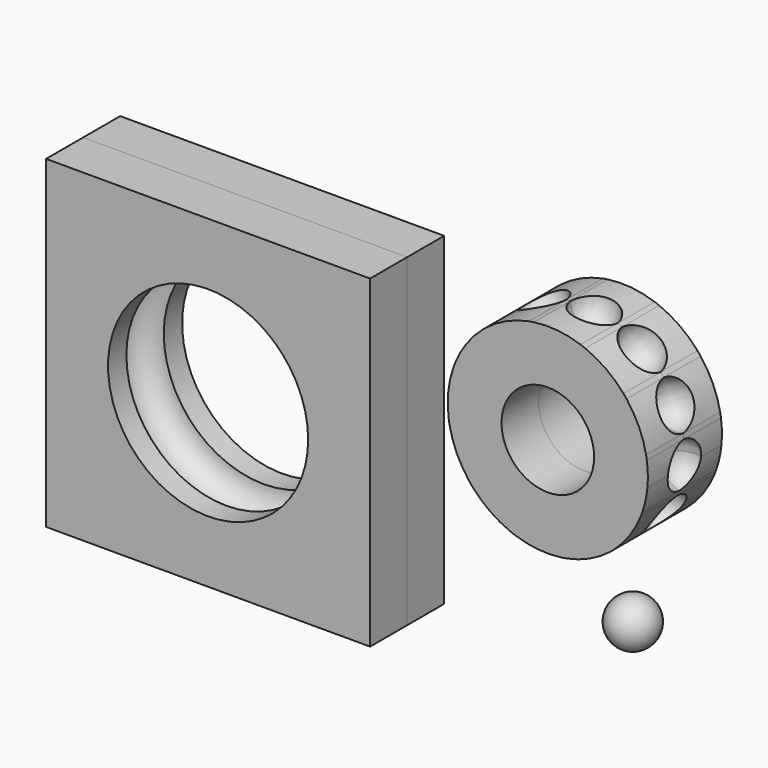
from build123d import *
from build123d import SkipClean  # not in build123d's __all__

# Parameters (mm, degrees)
F2_W      = 88.9
F2_H      = 88.9
F2_R      = 27.45
F5_DEPTH  = 12.7
F4_R      = 6.41
F7_R      = 12.7
F8_DEPTH  = 12.7
F22_W     = 3.2742018811
F22_H     = 5.4303631186
F23_DEPTH = 0.1
F22_R     = 2.7331759806
F24_DEPTH = 0.1


with BuildPart() as f1:
    # F0 (on Front) → F1 (revolve)
    with BuildSketch(Plane.XZ):
        with BuildLine():
            Line((0, 6.5), (0, -6.5))
            ThreePointArc((0, -6.5), (6.5, 0), (0, 6.5))
        make_face()
    revolve(axis=Axis((0, 0, 0), (0, 0, -1)))


with BuildPart() as f5:
    # F2 (on Front) → F5 (new body)
    with BuildSketch(Plane.XZ):
        with Locations((-106.35, 23.4373745618)):
            Rectangle(F2_W, F2_H)
        with Locations((-106.35, 23.4373745618)):
            Circle(F2_R, mode=Mode.SUBTRACT)
    extrude(amount=F5_DEPTH)

    # F4 (on face) → F6 (revolve, cut)
    with BuildSketch(Plane(origin=(0, 0, 23.4373745618), x_dir=(1, 0, 0), z_dir=(0, 0, -1))):
        with Locations((-133.8, 0)):
            Circle(F4_R)
    revolve(axis=Axis((-106.35, 0, 23.4373745618), (0, -1, 0)), mode=Mode.SUBTRACT)

    # F25: F5 across face


with BuildPart() as f8:
    # F7 (on Front) → F8 (new body)
    with BuildSketch(Plane.XZ):
        with BuildLine():
            Line((13.4063024508, 42.210689718), (14.0268309363, 48.6350721316))
            ThreePointArc((14.0268309363, 48.6350721316), (9.7490674331, 46.8995620632), (7.7024290215, 42.7616245336))
            Line((7.7024290215, 42.7616245336), (13.4063024508, 42.210689718))
        make_face()
        with BuildLine():
            Line((13.4063024508, 42.210689718), (7.7024290215, 42.7616245336))
            ThreePointArc((7.7024290215, 42.7616245336), (8.9192573509, 38.3084700783), (12.7857739652, 35.7863073044))
            Line((12.7857739652, 35.7863073044), (13.4063024508, 42.210689718))
        make_face()
        with BuildLine():
            ThreePointArc((14.1723185105, 42.1367005382), (14.2676693344, 43.4547207628), (14.2994775146, 44.7758026421))
            ThreePointArc((14.2994775146, 44.7758026421), (14.2312310325, 46.7102468225), (14.0268309363, 48.6350721316))
            Line((14.0268309363, 48.6350721316), (13.4063024508, 42.210689718))
            Line((13.4063024508, 42.210689718), (14.1723185105, 42.1367005382))
        make_face()
        with BuildLine():
            ThreePointArc((12.7857739652, 35.7863073044), (13.6676766328, 38.9203183702), (14.1723185105, 42.1367005382))
            Line((14.1723185105, 42.1367005382), (13.4063024508, 42.210689718))
            Line((13.4063024508, 42.210689718), (12.7857739652, 35.7863073044))
        make_face()
        with BuildLine():
            Line((8.4561212407, 61.7067047709), (13.8057167898, 49.9588195377))
            ThreePointArc((13.8057167898, 49.9588195377), (11.8313029726, 56.1516936749), (8.4561212407, 61.7067047709))
        make_face()
        with BuildLine():
            Line((-2.9040711925, 70.2417158577), (7.6027570696, 62.7425465795))
            ThreePointArc((7.6027570696, 62.7425465795), (2.7964274777, 67.1185259961), (-2.9040711925, 70.2417158577))
        make_face()
        with BuildLine():
            ThreePointArc((8.4561212407, 61.7067047709), (5.9157523177, 53.4579489859), (13.8057167898, 49.9588195377))
            Line((13.8057167898, 49.9588195377), (8.4561212407, 61.7067047709))
        make_face()
        with BuildLine():
            ThreePointArc((-2.9040711925, 70.2417158577), (-0.9797173223, 61.8278993367), (7.6027570696, 62.7425465795))
            Line((7.6027570696, 62.7425465795), (-2.9040711925, 70.2417158577))
        make_face()
        with BuildLine():
            ThreePointArc((-17.0097919748, 71.9531560638), (-11.1363443769, 65.628754149), (-4.1610271476, 70.7120990927))
            Line((-4.1610271476, 70.7120990927), (-17.0097919748, 71.9531560638))
        make_face()
        with BuildLine():
            ThreePointArc((-30.0814246141, 66.3824463682), (-21.8326688291, 63.8420774452), (-18.333539381, 71.7320419173))
            Line((-18.333539381, 71.7320419173), (-30.0814246141, 66.3824463682))
        make_face()
        with BuildLine():
            ThreePointArc((-38.6164357009, 55.022253935), (-30.20261918, 56.9466078052), (-31.1172664228, 65.5290821971))
            Line((-31.1172664228, 65.5290821971), (-38.6164357009, 55.022253935))
        make_face()
        with BuildLine():
            ThreePointArc((7.7024290215, 42.7616245336), (9.7490674331, 46.8995620632), (14.0268309363, 48.6350721316))
            ThreePointArc((14.0268309363, 48.6350721316), (13.9243651666, 49.2982973777), (13.8057167898, 49.9588195377))
            ThreePointArc((13.8057167898, 49.9588195377), (5.9157523177, 53.4579489859), (8.4561212407, 61.7067047709))
            ThreePointArc((8.4561212407, 61.7067047709), (8.035770658, 62.2298417976), (7.6027570696, 62.7425465795))
            ThreePointArc((7.6027570696, 62.7425465795), (-0.9797173223, 61.8278993367), (-2.9040711925, 70.2417158577))
            ThreePointArc((-2.9040711925, 70.2417158577), (-3.5296739889, 70.4845905211), (-4.1610271476, 70.7120990927))
            ThreePointArc((-4.1610271476, 70.7120990927), (-11.1363443769, 65.628754149), (-17.0097919748, 71.9531560638))
            ThreePointArc((-17.0097919748, 71.9531560638), (-17.673017221, 71.8506902941), (-18.333539381, 71.7320419173))
            ThreePointArc((-18.333539381, 71.7320419173), (-21.8326688291, 63.8420774452), (-30.0814246141, 66.3824463682))
            ThreePointArc((-30.0814246141, 66.3824463682), (-30.6045616409, 65.9620957855), (-31.1172664228, 65.5290821971))
            ThreePointArc((-31.1172664228, 65.5290821971), (-30.20261918, 56.9466078052), (-38.6164357009, 55.022253935))
            ThreePointArc((-38.6164357009, 55.022253935), (-38.8593103644, 54.3966511385), (-39.086818936, 53.7652979798))
            ThreePointArc((-39.086818936, 53.7652979798), (-34.0034739922, 46.7899807506), (-40.3278759071, 40.9165331526))
            ThreePointArc((-40.3278759071, 40.9165331526), (-40.2254101373, 40.2533079065), (-40.1067617605, 39.5927857465))
            ThreePointArc((-40.1067617605, 39.5927857465), (-32.2167972884, 36.0936562984), (-34.7571662115, 27.8449005133))
            ThreePointArc((-34.7571662115, 27.8449005133), (-34.3368156288, 27.3217634866), (-33.9038020403, 26.8090587047))
            ThreePointArc((-33.9038020403, 26.8090587047), (-25.3213276485, 27.7237059475), (-23.3969737783, 19.3098894266))
            ThreePointArc((-23.3969737783, 19.3098894266), (-22.7713709818, 19.0670147631), (-22.1400178231, 18.8395061915))
            ThreePointArc((-22.1400178231, 18.8395061915), (-15.1647005938, 23.9228511352), (-9.2912529959, 17.5984492204))
            ThreePointArc((-9.2912529959, 17.5984492204), (-8.6280277497, 17.7009149901), (-7.9675055898, 17.8195633669))
            ThreePointArc((-7.9675055898, 17.8195633669), (-4.4683761416, 25.7095278391), (3.7803796434, 23.169158916))
            ThreePointArc((3.7803796434, 23.169158916), (4.3035166702, 23.5895094987), (4.8162214521, 24.0225230871))
            ThreePointArc((4.8162214521, 24.0225230871), (3.9015742092, 32.604997479), (12.3153907302, 34.5293513492))
            ThreePointArc((12.3153907302, 34.5293513492), (12.5582653936, 35.1549541457), (12.7857739652, 35.7863073044))
            ThreePointArc((12.7857739652, 35.7863073044), (8.9192573509, 38.3084700783), (7.7024290215, 42.7616245336))
        make_face()
        with Locations((-13.1505224854, 44.7758026421)):
            Circle(F7_R, mode=Mode.SUBTRACT)
        with BuildLine():
            Line((4.8162214521, 24.0225230871), (12.3153907302, 34.5293513492))
            ThreePointArc((12.3153907302, 34.5293513492), (3.9015742092, 32.604997479), (4.8162214521, 24.0225230871))
        make_face()
        with BuildLine():
            Line((-7.9675055898, 17.8195633669), (3.7803796434, 23.169158916))
            ThreePointArc((3.7803796434, 23.169158916), (-4.4683761416, 25.7095278391), (-7.9675055898, 17.8195633669))
        make_face()
        with BuildLine():
            Line((-22.1400178231, 18.8395061915), (-9.2912529959, 17.5984492204))
            ThreePointArc((-9.2912529959, 17.5984492204), (-15.1647005938, 23.9228511352), (-22.1400178231, 18.8395061915))
        make_face()
        with BuildLine():
            Line((-33.9038020403, 26.8090587047), (-23.3969737783, 19.3098894266))
            ThreePointArc((-23.3969737783, 19.3098894266), (-25.3213276485, 27.7237059475), (-33.9038020403, 26.8090587047))
        make_face()
        with BuildLine():
            Line((-40.1067617605, 39.5927857465), (-34.7571662115, 27.8449005133))
            ThreePointArc((-34.7571662115, 27.8449005133), (-32.2167972884, 36.0936562984), (-40.1067617605, 39.5927857465))
        make_face()
        with BuildLine():
            ThreePointArc((-40.3278759071, 40.9165331526), (-34.0034739922, 46.7899807506), (-39.086818936, 53.7652979798))
            Line((-39.086818936, 53.7652979798), (-40.3278759071, 40.9165331526))
        make_face()
        with BuildLine():
            Line((-30.0814246141, 66.3824463682), (-18.333539381, 71.7320419173))
            ThreePointArc((-18.333539381, 71.7320419173), (-24.5264135181, 69.7576281), (-30.0814246141, 66.3824463682))
        make_face()
        with BuildLine():
            Line((-38.6164357009, 55.022253935), (-31.1172664228, 65.5290821971))
            ThreePointArc((-31.1172664228, 65.5290821971), (-35.4932458394, 60.7227526052), (-38.6164357009, 55.022253935))
        make_face()
        with BuildLine():
            Line((-17.0097919748, 71.9531560638), (-4.1610271476, 70.7120990927))
            ThreePointArc((-4.1610271476, 70.7120990927), (-10.5114203815, 72.098643638), (-17.0097919748, 71.9531560638))
        make_face()
        with BuildLine():
            Line((-40.3278759071, 40.9165331526), (-39.086818936, 53.7652979798))
            ThreePointArc((-39.086818936, 53.7652979798), (-40.4733634812, 47.414904746), (-40.3278759071, 40.9165331526))
        make_face()
        with BuildLine():
            ThreePointArc((-40.1067617605, 39.5927857465), (-38.1323479433, 33.3999116094), (-34.7571662115, 27.8449005133))
            Line((-34.7571662115, 27.8449005133), (-40.1067617605, 39.5927857465))
        make_face()
        with BuildLine():
            ThreePointArc((-33.9038020403, 26.8090587047), (-29.0974724485, 22.4330792881), (-23.3969737783, 19.3098894266))
            Line((-23.3969737783, 19.3098894266), (-33.9038020403, 26.8090587047))
        make_face()
        with BuildLine():
            ThreePointArc((-22.1400178231, 18.8395061915), (-15.7896245893, 17.4529616462), (-9.2912529959, 17.5984492204))
            Line((-9.2912529959, 17.5984492204), (-22.1400178231, 18.8395061915))
        make_face()
        with BuildLine():
            ThreePointArc((-7.9675055898, 17.8195633669), (-1.7746314526, 19.7939771842), (3.7803796434, 23.169158916))
            Line((3.7803796434, 23.169158916), (-7.9675055898, 17.8195633669))
        make_face()
        with BuildLine():
            ThreePointArc((4.8162214521, 24.0225230871), (9.1922008686, 28.828852679), (12.3153907302, 34.5293513492))
            Line((12.3153907302, 34.5293513492), (4.8162214521, 24.0225230871))
        make_face()
    extrude(amount=F8_DEPTH)

    # F7 (on Front) → F9 (revolve, cut)
    with BuildSketch(Plane.XZ):
        with BuildLine():
            Line((13.4063024508, 42.210689718), (14.0268309363, 48.6350721316))
            ThreePointArc((14.0268309363, 48.6350721316), (9.7490674331, 46.8995620632), (7.7024290215, 42.7616245336))
            Line((7.7024290215, 42.7616245336), (13.4063024508, 42.210689718))
        make_face()
        with BuildLine():
            Line((13.4063024508, 42.210689718), (7.7024290215, 42.7616245336))
            ThreePointArc((7.7024290215, 42.7616245336), (8.9192573509, 38.3084700783), (12.7857739652, 35.7863073044))
            Line((12.7857739652, 35.7863073044), (13.4063024508, 42.210689718))
        make_face()
    revolve(axis=Axis((13.4063024508, 0, 42.210689718), (-0.0961421531, 0, -0.9953676137)), mode=Mode.SUBTRACT)

    # F7 (on Front) → F10 (revolve, cut)
    with BuildSketch(Plane.XZ):
        with BuildLine():
            ThreePointArc((8.4561212407, 61.7067047709), (5.9157523177, 53.4579489859), (13.8057167898, 49.9588195377))
            Line((13.8057167898, 49.9588195377), (8.4561212407, 61.7067047709))
        make_face()
    revolve(axis=Axis((11.1309190152, 0, 55.8327621543), (0.4144222598, 0, -0.9100847161)), mode=Mode.SUBTRACT)

    # F7 (on Front) → F11 (revolve, cut)
    with BuildSketch(Plane.XZ):
        with BuildLine():
            ThreePointArc((-2.9040711925, 70.2417158577), (-0.9797173223, 61.8278993367), (7.6027570696, 62.7425465795))
            Line((7.6027570696, 62.7425465795), (-2.9040711925, 70.2417158577))
        make_face()
    revolve(axis=Axis((2.3493429386, 0, 66.4921312186), (0.813942563, 0, -0.5809453538)), mode=Mode.SUBTRACT)

    # F7 (on Front) → F12 (revolve, cut)
    with BuildSketch(Plane.XZ):
        with BuildLine():
            ThreePointArc((-17.0097919748, 71.9531560638), (-11.1363443769, 65.628754149), (-4.1610271476, 70.7120990927))
            Line((-4.1610271476, 70.7120990927), (-17.0097919748, 71.9531560638))
        make_face()
    revolve(axis=Axis((-10.5854095612, 0, 71.3326275782), (0.9953676137, 0, -0.0961421531)), mode=Mode.SUBTRACT)

    # F7 (on Front) → F13 (revolve, cut)
    with BuildSketch(Plane.XZ):
        with BuildLine():
            ThreePointArc((-30.0814246141, 66.3824463682), (-21.8326688291, 63.8420774452), (-18.333539381, 71.7320419173))
            Line((-18.333539381, 71.7320419173), (-30.0814246141, 66.3824463682))
        make_face()
    revolve(axis=Axis((-24.2074819976, 0, 69.0572441427), (0.9100847161, 0, 0.4144222598)), mode=Mode.SUBTRACT)

    # F7 (on Front) → F14 (revolve, cut)
    with BuildSketch(Plane.XZ):
        with BuildLine():
            ThreePointArc((-38.6164357009, 55.022253935), (-30.20261918, 56.9466078052), (-31.1172664228, 65.5290821971))
            Line((-31.1172664228, 65.5290821971), (-38.6164357009, 55.022253935))
        make_face()
    revolve(axis=Axis((-34.8668510619, 0, 60.2756680661), (0.5809453538, 0, 0.813942563)), mode=Mode.SUBTRACT)

    # F7 (on Front) → F15 (revolve, cut)
    with BuildSketch(Plane.XZ):
        with BuildLine():
            ThreePointArc((-40.3278759071, 40.9165331526), (-34.0034739922, 46.7899807506), (-39.086818936, 53.7652979798))
            Line((-39.086818936, 53.7652979798), (-40.3278759071, 40.9165331526))
        make_face()
    revolve(axis=Axis((-39.7073474215, 0, 47.3409155662), (0.0961421531, 0, 0.9953676137)), mode=Mode.SUBTRACT)

    # F7 (on Front) → F16 (revolve, cut)
    with BuildSketch(Plane.XZ):
        with BuildLine():
            Line((-40.1067617605, 39.5927857465), (-34.7571662115, 27.8449005133))
            ThreePointArc((-34.7571662115, 27.8449005133), (-32.2167972884, 36.0936562984), (-40.1067617605, 39.5927857465))
        make_face()
    revolve(axis=Axis((-37.431963986, 0, 33.7188431299), (-0.4144222598, 0, 0.9100847161)), mode=Mode.SUBTRACT)

    # F7 (on Front) → F17 (revolve, cut)
    with BuildSketch(Plane.XZ):
        with BuildLine():
            Line((-33.9038020403, 26.8090587047), (-23.3969737783, 19.3098894266))
            ThreePointArc((-23.3969737783, 19.3098894266), (-25.3213276485, 27.7237059475), (-33.9038020403, 26.8090587047))
        make_face()
    revolve(axis=Axis((-28.6503879093, 0, 23.0594740656), (-0.813942563, 0, 0.5809453538)), mode=Mode.SUBTRACT)

    # F7 (on Front) → F18 (revolve, cut)
    with BuildSketch(Plane.XZ):
        with BuildLine():
            Line((-22.1400178231, 18.8395061915), (-9.2912529959, 17.5984492204))
            ThreePointArc((-9.2912529959, 17.5984492204), (-15.1647005938, 23.9228511352), (-22.1400178231, 18.8395061915))
        make_face()
    revolve(axis=Axis((-15.7156354095, 0, 18.218977706), (-0.9953676137, 0, 0.0961421531)), mode=Mode.SUBTRACT)

    # F7 (on Front) → F19 (revolve, cut)
    with BuildSketch(Plane.XZ):
        with BuildLine():
            Line((-7.9675055898, 17.8195633669), (3.7803796434, 23.169158916))
            ThreePointArc((3.7803796434, 23.169158916), (-4.4683761416, 25.7095278391), (-7.9675055898, 17.8195633669))
        make_face()
    revolve(axis=Axis((-2.0935629732, 0, 20.4943611415), (-0.9100847161, 0, -0.4144222598)), mode=Mode.SUBTRACT)

    # F7 (on Front) → F20 (revolve, cut)
    with BuildSketch(Plane.XZ):
        with BuildLine():
            Line((4.8162214521, 24.0225230871), (12.3153907302, 34.5293513492))
            ThreePointArc((12.3153907302, 34.5293513492), (3.9015742092, 32.604997479), (4.8162214521, 24.0225230871))
        make_face()
    revolve(axis=Axis((8.5658060911, 0, 29.2759372182), (-0.5809453538, 0, -0.813942563)), mode=Mode.SUBTRACT)

    # F21: F8 across face


with BuildPart() as f8_1:
    add(f8.part, clean=False)
    add(f8.part.mirror(Plane(origin=(-13.1505224854, 0, 44.7758026421), x_dir=(1, 0, 0), z_dir=(0, 1, 0))), clean=False)

    # F22 (on face) → F23 (cut)
    with BuildSketch(Plane(origin=(0, 12.7, 0), x_dir=(-1, 0, 0), z_dir=(0, 1, 0))):
        with Locations((-6.9112211931, 44.7133220732)):
            Rectangle(F22_W, F22_H)
    extrude(amount=-F23_DEPTH, mode=Mode.SUBTRACT)

    # F22 (on face) → F24 (cut)
    with BuildSketch(Plane(origin=(0, 12.7, 0), x_dir=(-1, 0, 0), z_dir=(0, 1, 0))):
        with Locations((32.5955525041, 42.0405752957)):
            Circle(F22_R)
    extrude(amount=-F24_DEPTH, mode=Mode.SUBTRACT)


with BuildPart() as f5_1:
    add(f5.part, clean=False)
    with SkipClean():  # cleaning this boolean's faces spoils the solid; the shape is the same uncleaned
        add(f5.part.mirror(Plane.XZ), clean=False)


solid = Compound([f1.part, f8_1.part, f5_1.part])
